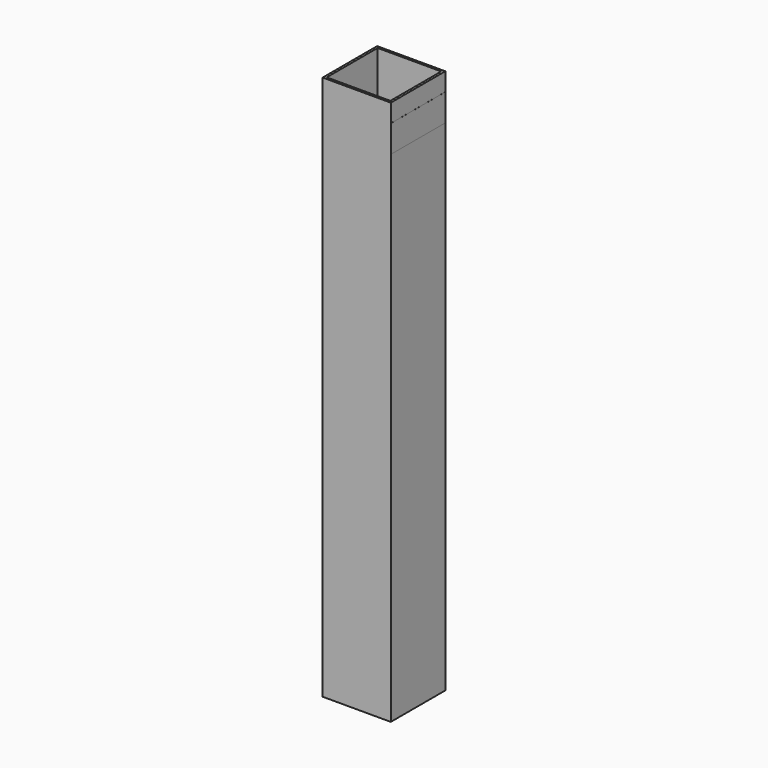
from build123d import *

# Parameters (mm, degrees)
F0_W     = 15
F0_H     = 15
F0_W_2   = 14
F0_H_2   = 14
F1_DEPTH = 60
F2_W     = 15
F2_H     = 6
F3_DEPTH = 0.01
F4_DEPTH = 60


with BuildPart() as f1:
    # F0 (on Top) → F1 (new body)
    with BuildSketch(Plane.XY):
        Rectangle(F0_W, F0_H)
        Rectangle(F0_W_2, F0_H_2, mode=Mode.SUBTRACT)
    extrude(amount=-F1_DEPTH)

    # F2 (on face) → F3 (join)
    with BuildSketch(Plane.YZ.offset(7.5)):
        with Locations((0, -7)):
            Rectangle(F2_W, F2_H)
    extrude(amount=F3_DEPTH)

    # F4 (add): a face of the model
    f4_faces = [f1.faces().sort_by_distance(p)[0] for p in [
        (0, -7.2878679656, -60),
    ]]
    extrude(f4_faces, amount=F4_DEPTH)


solid = f1.part
